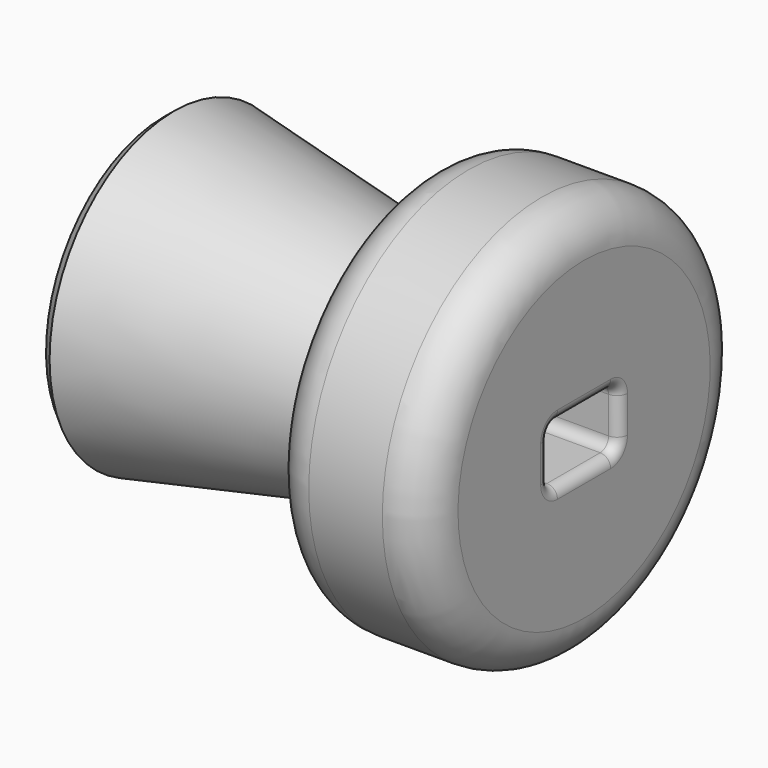
from build123d import *

# Parameters (mm, degrees)
F2_W     = 8.328109514
F2_H     = 5.4839188233
F3_DEPTH = 40.001
F4_SIZE  = 1
F5_F1_R  = 1
F5_F2_R  = 1
F5_F3_R  = 1


with BuildPart() as f1:
    # F0 (on Front) → F1 (revolve)
    with BuildSketch(Plane.XZ):
        with BuildLine():
            Line((0, 15), (0, 0))
            Line((0, 0), (40, 0))
            Line((40, 0), (40, 15))
            ThreePointArc((40, 15), (38.8284271247, 17.8284271247), (36, 19))
            Line((36, 19), (29, 19))
            ThreePointArc((29, 19), (26.1715728753, 17.8284271247), (25, 15))
            Line((25, 15), (25, 10))
            Line((25, 10), (0, 15))
        make_face()
    revolve(axis=Axis((20, 0, 0), (-1, 0, 0)))

    # F2 (on face) → F3 (cut, through all)
    with BuildSketch(Plane(origin=(0, 0, 0), x_dir=(0, -1, 0), z_dir=(-1, 0, 0))):
        Rectangle(F2_W, F2_H)
    extrude(amount=-F3_DEPTH, mode=Mode.SUBTRACT)

    # F4
    f4_edges = [f1.edges().sort_by_distance(p)[0] for p in [
        (0, 0, -15),
    ]]
    chamfer(f4_edges, length=F4_SIZE)

    # F5: fillet of radius 1 on 8 edges, made by hand

    # F5_f1
    f5_f1_edges = [f1.edges().sort_by_distance(p)[0] for p in [
        (20, -4.164054757, 2.7419594117),
        (20, -4.164054757, -2.7419594117),
        (20, 4.164054757, 2.7419594117),
        (20, 4.164054757, -2.7419594117),
    ]]
    fillet(f5_f1_edges, radius=F5_F1_R)

    # F5_f2
    f5_f2_edges = [f1.edges().sort_by_distance(p)[0] for p in [
        (0, -4.164054757, 0),
        (0, 4.164054757, 0),
        (0, 3.8711615382, 2.4490661928),
        (0, 3.8711615382, -2.4490661928),
        (0, -3.8711615382, -2.4490661928),
        (0, -3.8711615382, 2.4490661928),
    ]]
    fillet(f5_f2_edges, radius=F5_F2_R)

    # F5_f3
    f5_f3_edges = [f1.edges().sort_by_distance(p)[0] for p in [
        (40, -4.164054757, 0),
        (40, 0, -2.7419594117),
        (40, -3.8711615382, -2.4490661928),
        (40, 3.8711615382, -2.4490661928),
        (40, -3.8711615382, 2.4490661928),
    ]]
    fillet(f5_f3_edges, radius=F5_F3_R)


solid = f1.part
